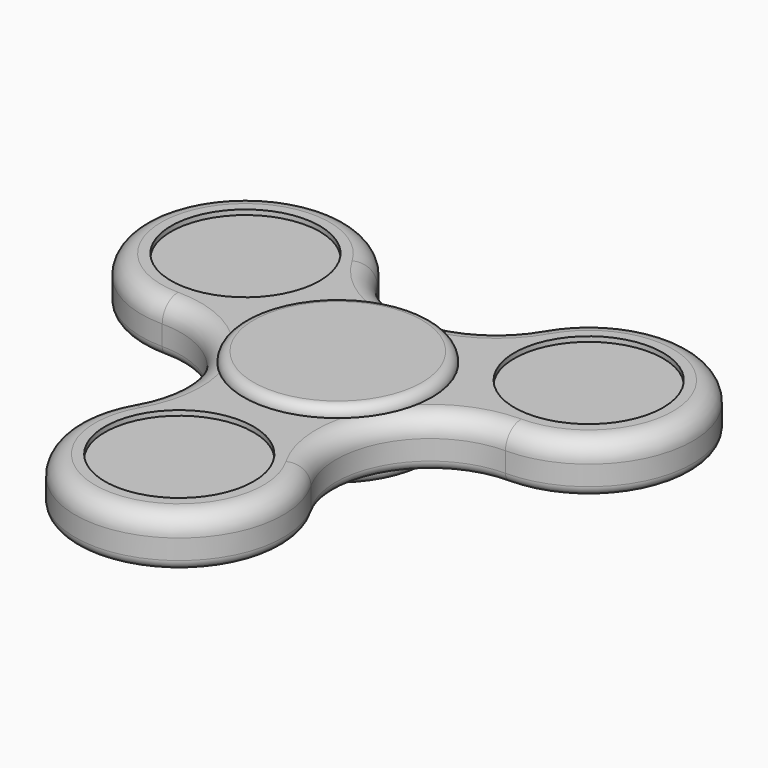
from build123d import *

# Parameters (mm, degrees)
F0_R     = 7.5
F1_DEPTH = 2.5
F2_DEPTH = 2
F3_R     = 7.4
F3_R_2   = 3
F4_DEPTH = 5.1
F3_R_3   = 9.5
F5_DEPTH = 1
F6_R     = 2.9
F7_DEPTH = 4.6
F6_R_2   = 9.5
F6_R_3   = 7.4
F6_R_4   = 3
F8_DEPTH = 1
F9_R     = 2
F10_R    = 0.99999
F11_R    = 0.99999
F11_2_R  = 0.99999


# Not quite as in the source:
# - a fillet or chamfer is up to 0.001 mm smaller than in the source, because OpenCascade refuses the exact size


with BuildPart() as f1:
    # F0 (on Top) → F1 (new body, symmetric)
    with BuildSketch(Plane.XY):
        with BuildLine():
            ThreePointArc((-17.3205080757, -0.5), (-9.0932667397, -5.25), (-9.0932667397, -14.75))
            ThreePointArc((-9.0932667397, -14.75), (0, -30.5), (9.0932667397, -14.75))
            ThreePointArc((9.0932667397, -14.75), (9.0932667397, -5.25), (17.3205080757, -0.5))
            ThreePointArc((17.3205080757, -0.5), (26.4137748154, 15.25), (8.227241336, 15.25))
            ThreePointArc((8.227241336, 15.25), (0, 10.5), (-8.227241336, 15.25))
            ThreePointArc((-8.227241336, 15.25), (-26.4137748154, 15.25), (-17.3205080757, -0.5))
        make_face()
        with Locations((0, -20)):
            Circle(F0_R, mode=Mode.SUBTRACT)
        with Locations((-17.3205080757, 10)):
            Circle(F0_R, mode=Mode.SUBTRACT)
        Circle(F0_R, mode=Mode.SUBTRACT)
        with Locations((17.3205080757, 10)):
            Circle(F0_R, mode=Mode.SUBTRACT)
    extrude(amount=F1_DEPTH, both=True)

    # F0 (on Top) → F2 (join, symmetric)
    with BuildSketch(Plane.XY):
        with Locations((0, -20)):
            Circle(F0_R)
        with Locations((17.3205080757, 10)):
            Circle(F0_R)
        with Locations((-17.3205080757, 10)):
            Circle(F0_R)
    extrude(amount=F2_DEPTH, both=True)

    # F9
    f9_edges = [f1.edges().sort_by_distance(p)[0] for p in [
        (-26.413775, 15.25, 2.5),
        (-9.093267, -5.25, 2.5),
        (0, -30.5, 2.5),
        (9.093267, -5.25, 2.5),
        (26.413775, 15.25, 2.5),
        (0, 10.5, 2.5),
    ]]
    fillet(f9_edges, radius=F9_R)

    # F11 (radius 1 in the source; OpenCascade refuses exactly that, so slightly less here)
    f11_edges = [f1.edges().sort_by_distance(p)[0] for p in [
        (-26.413775, 15.25, -2.5),
        (-9.093267, -5.25, -2.5),
        (0, -30.5, -2.5),
        (9.093267, -5.25, -2.5),
        (26.413775, 15.25, -2.5),
        (0, 10.5, -2.5),
    ]]
    fillet(f11_edges, radius=F11_R)


with BuildPart() as f4:
    # F3 (on face) → F4 (new body)
    with BuildSketch(Plane.XY.offset(2.5)):
        Circle(F3_R)
        Circle(F3_R_2, mode=Mode.SUBTRACT)
    extrude(amount=-F4_DEPTH)

    # F3 (on face) → F5 (join)
    with BuildSketch(Plane.XY.offset(2.5)):
        Circle(F3_R_3)
        Circle(F3_R, mode=Mode.SUBTRACT)
        Circle(F3_R)
        Circle(F3_R_2, mode=Mode.SUBTRACT)
        Circle(F3_R_2)
    extrude(amount=F5_DEPTH)

    # F10 (radius 1 in the source; OpenCascade refuses exactly that, so slightly less here)
    f10_edges = [f4.edges().sort_by_distance(p)[0] for p in [
        (-9.5, 0, 3.5),
    ]]
    fillet(f10_edges, radius=F10_R)


with BuildPart() as f7:
    # F6 (on face) → F7 (new body, through all)
    with BuildSketch(Plane(origin=(0, 0, -2.6), x_dir=(1, 0, 0), z_dir=(0, 0, -1))):
        Circle(F6_R)
    extrude(amount=-F7_DEPTH)

    # F6 (on face) → F8 (join)
    with BuildSketch(Plane(origin=(0, 0, -2.6), x_dir=(1, 0, 0), z_dir=(0, 0, -1))):
        Circle(F6_R_2)
        Circle(F6_R_3, mode=Mode.SUBTRACT)
        Circle(F6_R_3)
        Circle(F6_R_4, mode=Mode.SUBTRACT)
        Circle(F6_R_4)
        Circle(F6_R, mode=Mode.SUBTRACT)
        Circle(F6_R)
    extrude(amount=F8_DEPTH)

    # F11#2 (radius 1 in the source; OpenCascade refuses exactly that, so slightly less here)
    f11_2_edges = [f7.edges().sort_by_distance(p)[0] for p in [
        (-9.5, 0, -3.6),
    ]]
    fillet(f11_2_edges, radius=F11_2_R)


solid = Compound([f1.part, f4.part, f7.part])
